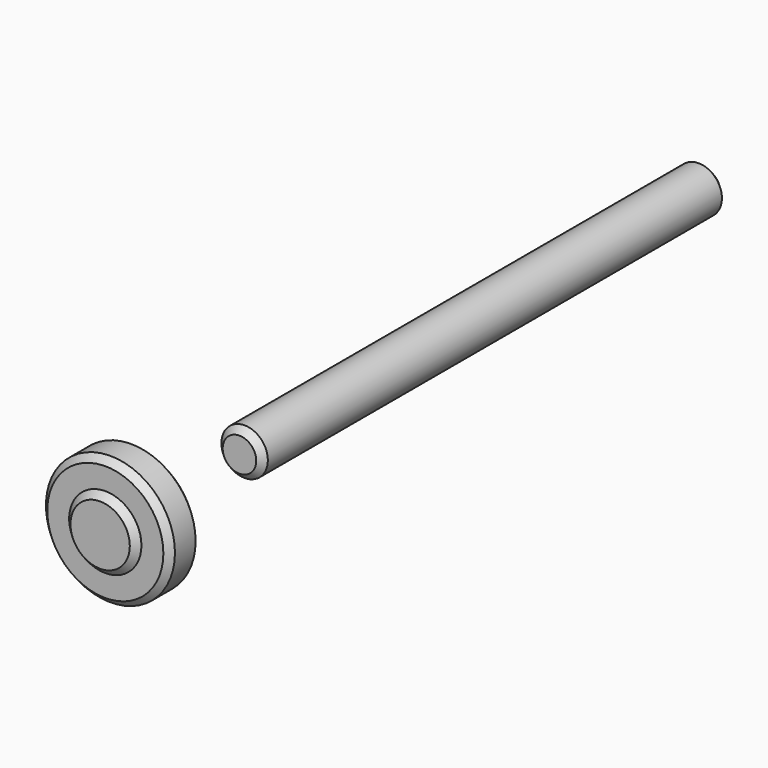
from build123d import *

# Parameters (mm, degrees)
F0_R     = 5
F0_R_2   = 2.8
F1_DEPTH = 3
F0_R_3   = 2
F0_R_4   = 1.8
F2_DEPTH = 3.5
F3_DEPTH = 2
F4_SIZE  = 0.49999
F5_START = -10
F5_DEPTH = 45
F6_SIZE  = 0.5


# Not quite as in the source:
# - a fillet or chamfer is up to 0.001 mm smaller than in the source, because OpenCascade refuses the exact size


with BuildPart() as f1:
    # F0 (on Front) → F1 (new body)
    with BuildSketch(Plane.XZ):
        Circle(F0_R)
        Circle(F0_R_2, mode=Mode.SUBTRACT)
    extrude(amount=F1_DEPTH)

    # F0 (on Front) → F2 (join)
    with BuildSketch(Plane.XZ):
        Circle(F0_R_2)
        Circle(F0_R_3, mode=Mode.SUBTRACT)
        Circle(F0_R_3)
        Circle(F0_R_4, mode=Mode.SUBTRACT)
        Circle(F0_R_4)
    extrude(amount=F2_DEPTH)

    # F0 (on Front) → F3 (cut)
    with BuildSketch(Plane.XZ):
        Circle(F0_R_3)
        Circle(F0_R_4, mode=Mode.SUBTRACT)
        Circle(F0_R_4)
    extrude(amount=F3_DEPTH, mode=Mode.SUBTRACT)

    # F4 (size 0.5 in the source; OpenCascade refuses exactly that, so slightly less here)
    f4_edges = [f1.edges().sort_by_distance(p)[0] for p in [
        (-2.8, -3.5, 0),
        (-5, -3, 0),
        (-5, 0, 0),
    ]]
    chamfer(f4_edges, length=F4_SIZE)


with BuildPart() as f5:
    # F0 (on Front) → F5 (new body)
    with BuildSketch(Plane.XZ.offset(F5_START)):
        Circle(F0_R_4)
    extrude(amount=-F5_DEPTH)

    # F6
    f6_edges = [f5.edges().sort_by_distance(p)[0] for p in [
        (-1.8, 55, 0),
        (-1.8, 10, 0),
    ]]
    chamfer(f6_edges, length=F6_SIZE)


solid = Compound([f1.part, f5.part])
